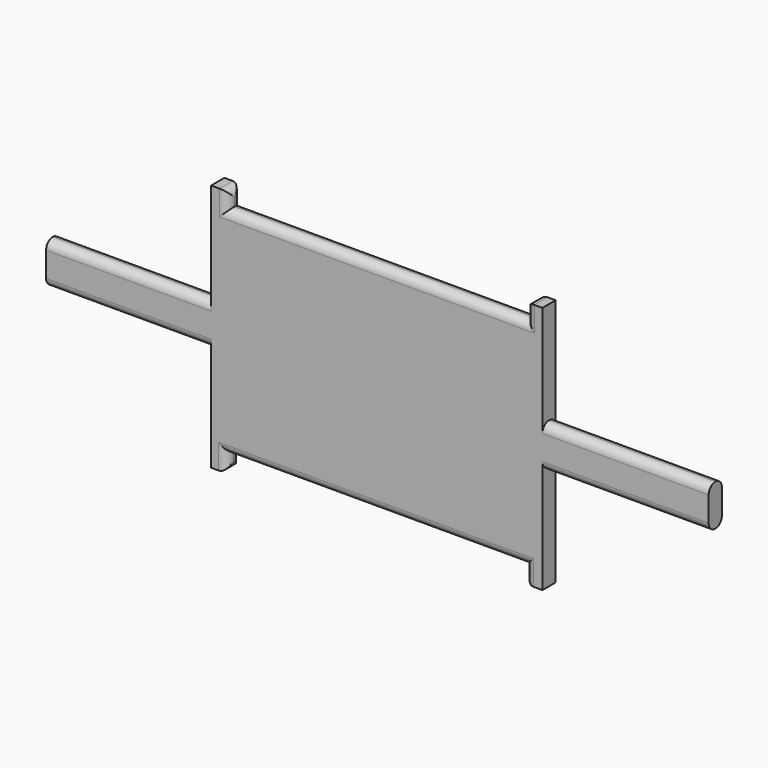
from build123d import *

# Parameters (mm, degrees)
F0_W     = 40
F0_H     = 5
F0_W_2   = 20.0747972727
F0_W_3   = 19.9252027273
F1_DEPTH = 2
F2_R     = 0.99999
F3_R     = 0.99999
F4_R     = 0.99999


# Not quite as in the source:
# - a fillet or chamfer is up to 0.001 mm smaller than in the source, because OpenCascade refuses the exact size


with BuildPart() as f1:
    # F0 (on Front) → F1 (new body)
    with BuildSketch(Plane.XZ):
        Polygon((-17.9821681231, 15), (-20, 15), (-20, 2.6505640079), (20, 2.6505640079), (20, 15), (18.0178318769, 15), (18.0178318769, 13), (-17.9821681231, 13), align=None)
        with Locations((0, 0.1505640079)):
            Rectangle(F0_W, F0_H)
        with Locations((30.0373986363, 0.1505640079)):
            Rectangle(F0_W_2, F0_H)
        with Locations((-29.9626013637, 0.1505640079)):
            Rectangle(F0_W_3, F0_H)
        Polygon((20, -2.3494359921), (-20, -2.3494359921), (-20, -15), (-18.0797521025, -15), (-18.0797521025, -13), (17.9202478975, -13), (17.9202478975, -15), (20, -15), align=None)
    extrude(amount=F1_DEPTH)

    # F2 (radius 1 in the source; OpenCascade refuses exactly that, so slightly less here)
    f2_edges = [f1.edges().sort_by_distance(p)[0] for p in [
        (30.037399, -2, -2.349436),
        (30.037399, 0, -2.349436),
        (30.037399, -2, 2.650564),
        (-29.962601, 0, 2.650564),
        (-29.962601, -2, 2.650564),
        (-29.962601, 0, -2.349436),
        (30.037399, 0, 2.650564),
        (-29.962601, -2, -2.349436),
    ]]
    fillet(f2_edges, radius=F2_R)

    # F3 (radius 1 in the source; OpenCascade refuses exactly that, so slightly less here)
    f3_edges = [f1.edges().sort_by_distance(p)[0] for p in [
        (-0.079752, -2, -13),
        (-0.079752, 0, -13),
        (0.017832, 0, 13),
        (0.017832, -2, 13),
    ]]
    fillet(f3_edges, radius=F3_R)

    # F4 (radius 1 in the source; OpenCascade refuses exactly that, so slightly less here)
    f4_edges = [f1.edges().sort_by_distance(p)[0] for p in [
        (18.017832, -2, 14),
        (18.017832, -1, 15),
        (18.017832, 0, 14),
        (-17.982168, -2, 14),
        (-17.982168, -1, 15),
        (-18.079752, -2, -14),
        (17.920248, -2, -14),
        (-17.982168, 0, 14),
        (-18.079752, 0, -14),
        (-18.079752, -1, -15),
        (17.920248, 0, -14),
        (17.920248, -1, -15),
    ]]
    fillet(f4_edges, radius=F4_R)


solid = f1.part
